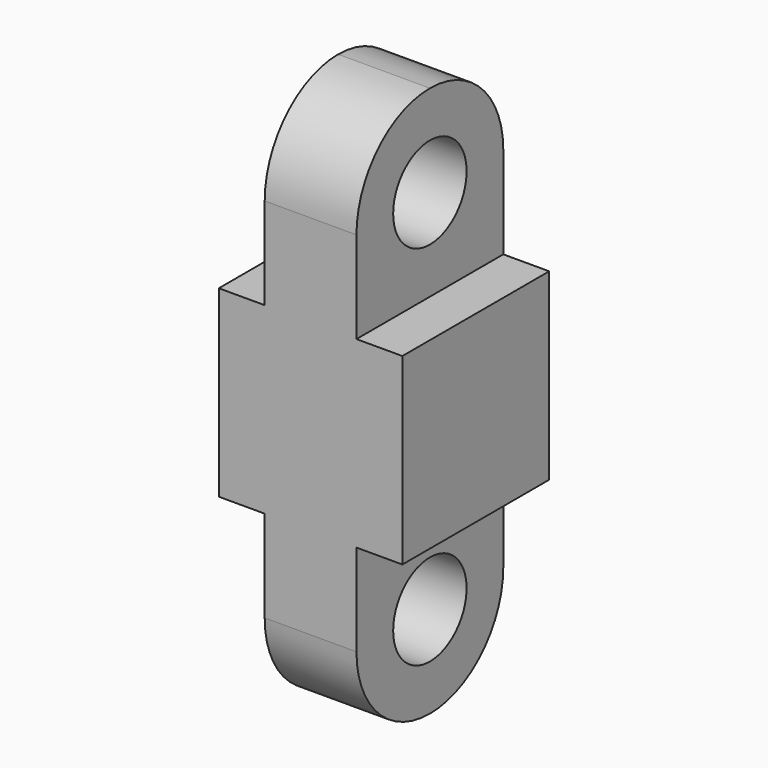
from build123d import *

# Parameters (mm, degrees)
F1_DEPTH = 40
F2_R     = 19.99999
F3_R     = 19.99999
F4_R     = 10
F5_DEPTH = 20
F6_R     = 10
F7_DEPTH = 20


# Not quite as in the source:
# - a fillet or chamfer is up to 0.001 mm smaller than in the source, because OpenCascade refuses the exact size


with BuildPart() as f1:
    # F0 (on Front) → F1 (new body)
    with BuildSketch(Plane.XZ):
        Polygon((3.91200836, 0), (23.91200836, 0), (23.91200836, 40), (33.91200836, 40), (33.91200836, 80), (23.91200836, 80), (23.91200836, 120), (3.91200836, 120), (3.91200836, 80), (-6.08799164, 80), (-6.08799164, 40), (3.91200836, 40), align=None)
    extrude(amount=F1_DEPTH)

    # F2 (radius 20 in the source; OpenCascade refuses exactly that, so slightly less here)
    f2_edges = [f1.edges().sort_by_distance(p)[0] for p in [
        (13.912008, 0, 120),
        (13.912008, -40, 120),
    ]]
    fillet(f2_edges, radius=F2_R)

    # F3 (radius 20 in the source; OpenCascade refuses exactly that, so slightly less here)
    f3_edges = [f1.edges().sort_by_distance(p)[0] for p in [
        (13.912008, -40, 0),
        (13.912008, 0, 0),
    ]]
    fillet(f3_edges, radius=F3_R)

    # F4 (on face) → F5 (cut, through all)
    with BuildSketch(Plane(origin=(3.91200836, 0, 0), x_dir=(0, -1, 0), z_dir=(-1, 0, 0))):
        with Locations((20, 100)):
            Circle(F4_R)
    extrude(amount=-F5_DEPTH, mode=Mode.SUBTRACT)

    # F6 (on face) → F7 (cut, through all)
    with BuildSketch(Plane(origin=(3.91200836, 0, 0), x_dir=(0, -1, 0), z_dir=(-1, 0, 0))):
        with Locations((20, 20)):
            Circle(F6_R)
    extrude(amount=-F7_DEPTH, mode=Mode.SUBTRACT)


solid = f1.part
